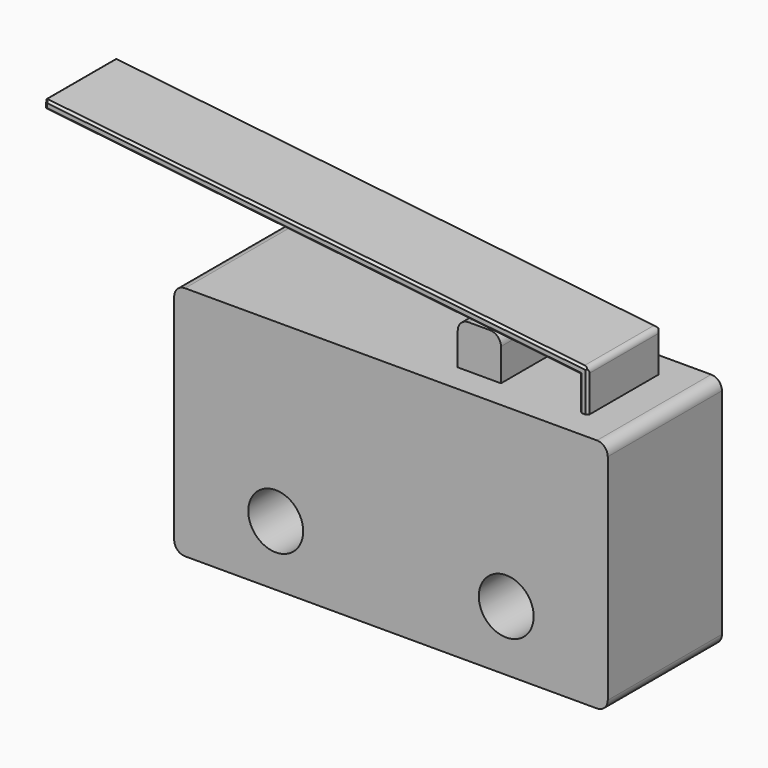
from build123d import *

# Parameters (mm, degrees)
F0_W     = 20.066
F0_H     = 10.922
F0_R     = 1.27
F1_DEPTH = 6.604
F2_W     = 2
F2_H     = 4.064
F3_DEPTH = 2
F4_R     = 0.5
F7_DEPTH = 4.2
F8_SIZE  = 0.1
F9_SIZE  = 0.19999
F10_R    = 0.25


# Not quite as in the source:
# - a fillet or chamfer is up to 0.001 mm smaller than in the source, because OpenCascade refuses the exact size


with BuildPart() as f1:
    # F0 (on Front) → F1 (new body)
    with BuildSketch(Plane.XZ):
        with Locations((10.033, -5.461)):
            Rectangle(F0_W, F0_H)
        with Locations((4.699, -8.128)):
            Circle(F0_R, mode=Mode.SUBTRACT)
        with Locations((15.367, -8.128)):
            Circle(F0_R, mode=Mode.SUBTRACT)
    extrude(amount=F1_DEPTH)

    # F2 (on face) → F3 (join)
    with BuildSketch(Plane.XY):
        with Locations((13.066, -3.2510236964)):
            Rectangle(F2_W, F2_H)
    extrude(amount=F3_DEPTH)

    # F4
    f4_edges = [f1.edges().sort_by_distance(p)[0] for p in [
        (12.066, -3.251024, 2),
        (14.066, -3.251024, 2),
        (0, -3.302, 0),
        (20.066, -3.302, 0),
        (0, -3.302, -10.922),
        (20.066, -3.302, -10.922),
    ]]
    fillet(f4_edges, radius=F4_R)


with BuildPart() as f7:
    # F6 (on face) → F7 (new body)
    with BuildSketch(Plane.XZ.offset(5.2830236964)):
        Polygon((18.0865991861, 0), (18.0865991861, 1.5), (17.6965991861, 1.5434021702), (17.6965991861, 0), align=None)
        Polygon((17.6965991861, 1.5434021702), (18.0865991861, 1.5), (18.0865991861, 1.9024693645), (-7.1133163265, 4.7069078814), (-7.1575582493, 4.309362095), (13.6213023921, 1.9969322342), align=None)
    extrude(amount=-F7_DEPTH)

    # F8
    f8_edges = [f7.edges().sort_by_distance(p)[0] for p in [
        (18.086599, -5.283024, 0.951235),
        (5.486641, -5.283024, 3.304689),
        (5.26952, -5.283024, 2.926382),
        (17.696599, -5.283024, 0.771701),
        (18.086599, -1.083024, 0.951235),
        (5.486641, -1.083024, 3.304689),
        (17.696599, -1.083024, 0.771701),
        (5.26952, -1.083024, 2.926382),
        (-7.113316, -3.183024, 4.706908),
        (-7.157558, -3.183024, 4.309362),
    ]]
    chamfer(f8_edges, length=F8_SIZE)

    # F9 (size 0.2 in the source; OpenCascade refuses exactly that, so slightly less here)
    f9_edges = [f7.edges().sort_by_distance(p)[0] for p in [
        (-7.135437, -5.283024, 4.508135),
        (-7.135437, -1.083024, 4.508135),
    ]]
    chamfer(f9_edges, length=F9_SIZE)

    # F10
    f10_edges = [f7.edges().sort_by_distance(p)[0] for p in [
        (17.696599, -3.183024, 1.543402),
        (18.086599, -3.183024, 1.902469),
    ]]
    fillet(f10_edges, radius=F10_R)


solid = Compound([f1.part, f7.part])
